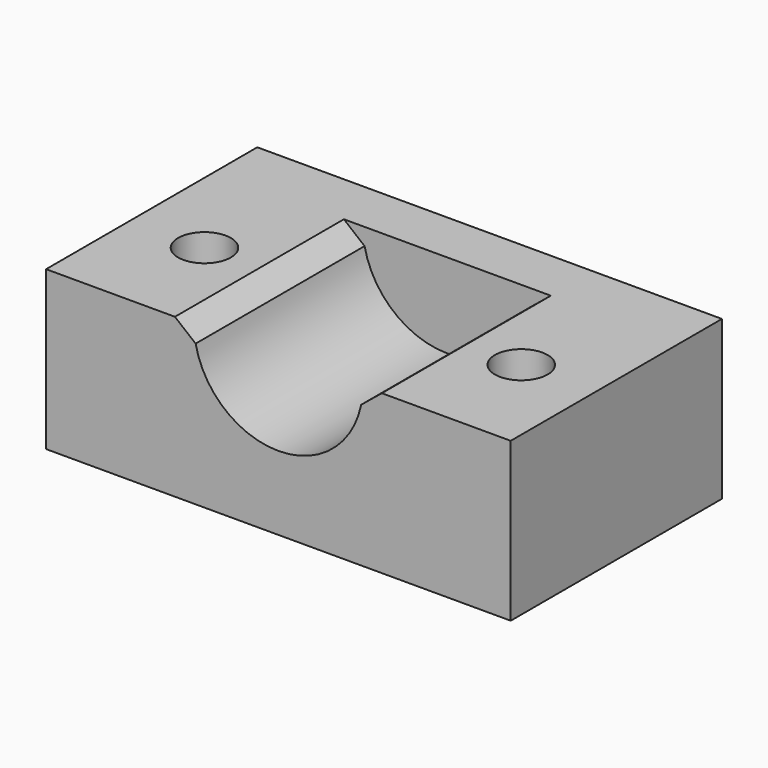
from build123d import *

# Parameters (mm, degrees)
F0_W        = 44
F0_H        = 25
F1_DEPTH    = 15
F2_R        = 8
F3_DEPTH    = 20
F4_R        = 2.5
F5_DEPTH    = 15
F6_T1_DEPTH = 24.6515369414


# Not quite as in the source:
# - a fillet or chamfer that OpenCascade refuses, or shapes differently, is made with other operations: its cross-section is extruded or revolved along the edge and cut away or added


with BuildPart() as f1:
    # F0 (on Top) → F1 (new body)
    with BuildSketch(Plane.XY):
        Rectangle(F0_W, F0_H)
    extrude(amount=F1_DEPTH)

    # F2 (on face) → F3 (cut)
    with BuildSketch(Plane.XZ.offset(12.5)):
        with Locations((0, 15)):
            Circle(F2_R)
    extrude(amount=-F3_DEPTH, mode=Mode.SUBTRACT)

    # F4 (on face) → F5 (cut)
    with BuildSketch(Plane.XY.offset(15)):
        with Locations((-15, -2.5)):
            Circle(F4_R)
        with Locations((15, -2.5)):
            Circle(F4_R)
    extrude(amount=-F5_DEPTH, mode=Mode.SUBTRACT)

    # F6: chamfer of 2 on 2 edges, made by hand

    # F6_s2 → F6_t1 (cut)
    with BuildSketch(Plane.XZ.offset(-7.5)):
        with BuildLine():
            Line((9.7979589711, 15), (7.8383671769, 13.4))
            ThreePointArc((7.8383671769, 13.4), (7.9565711479, 14.1675484588), (8, 15))
            Line((8, 15), (9.7979589711, 15))
        make_face()
        with BuildLine():
            Line((-9.7979589711, 15), (-7.8383671769, 13.4))
            ThreePointArc((-7.8383671769, 13.4), (-7.9565711479, 14.1675484588), (-8, 15))
            Line((-8, 15), (-9.7979589711, 15))
        make_face()
    extrude(amount=F6_T1_DEPTH, mode=Mode.SUBTRACT)


solid = f1.part
